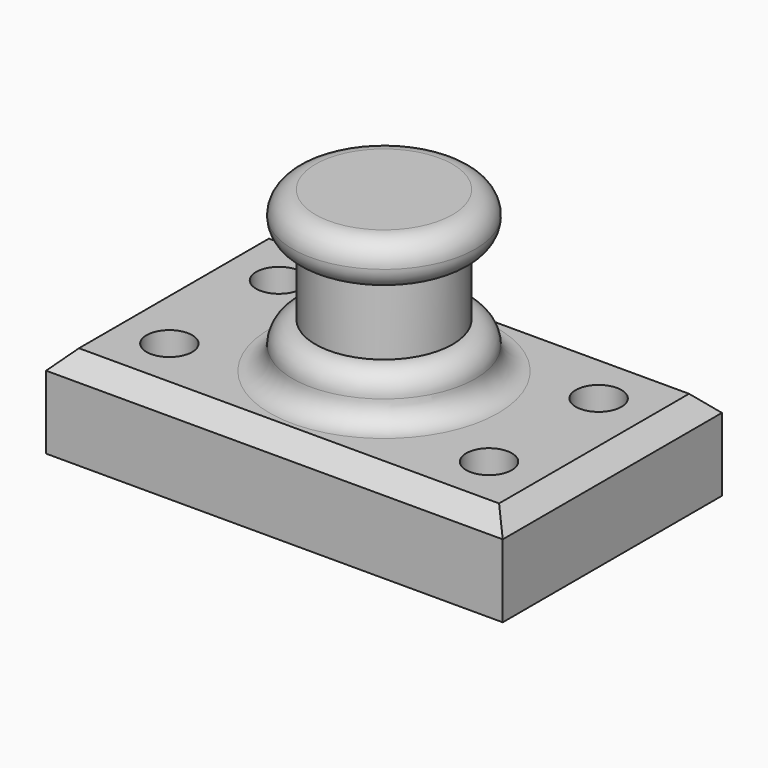
from build123d import *

# Parameters (mm, degrees)
F1_DEPTH = 25.4
F2_R     = 6.35
F3_DEPTH = 25.4
F4_W     = 25.4
F4_H     = 12.7
F6_W     = 19.05
F6_H     = 19.05
F8_W     = 25.4
F8_H     = 12.7
F11_R    = 6.34999
F12_SIZE = 5.08


# Not quite as in the source:
# - a fillet or chamfer is up to 0.001 mm smaller than in the source, because OpenCascade refuses the exact size
# - a feature of the source that left no trace in its solid (it failed there, or was rolled back) is left out


with BuildPart() as f1:
    # F0 (on Top) → F1 (new body)
    with BuildSketch(Plane.XY):
        Polygon((-63.0538856602, 38.1), (-63.5, 38.1), (-63.5, -38.1), (63.5, -38.1), (63.5, 38.1), align=None)
    extrude(amount=F1_DEPTH)

    # F2 (on face) → F3 (cut)
    with BuildSketch(Plane.XY.offset(25.4)):
        with Locations((-44.45, 19.05)):
            Circle(F2_R)
        with Locations((-44.45, -19.05)):
            Circle(F2_R)
        with Locations((44.45, 19.05)):
            Circle(F2_R)
        with Locations((44.45, -19.05)):
            Circle(F2_R)
    extrude(amount=-F3_DEPTH, mode=Mode.SUBTRACT)

    # F4 (on Front) → F5 (revolve)
    with BuildSketch(Plane.XZ):
        with Locations((12.7, 31.75)):
            Rectangle(F4_W, F4_H)
    revolve(axis=Axis((0, 0, 31.75), (0, 0, -1)))

    # F6 (on Front) → F7 (revolve)
    with BuildSketch(Plane.XZ):
        with Locations((9.525, 47.625)):
            Rectangle(F6_W, F6_H)
    revolve(axis=Axis((0, 0, 47.625), (0, 0, 1)))

    # F8 (on Front) → F9 (revolve)
    with BuildSketch(Plane.XZ):
        with Locations((12.7, 63.5)):
            Rectangle(F8_W, F8_H)
    revolve(axis=Axis((0, 0, 63.5), (0, 0, 1)))

    # F11 (radius 6.35 in the source; OpenCascade refuses exactly that, so slightly less here)
    f11_edges = [f1.edges().sort_by_distance(p)[0] for p in [
        (-25.4, 0, 69.85),
        (-25.4, 0, 38.1),
        (-25.4, 0, 57.15),
        (-25.4, 0, 25.4),
        (25.4, 0, 31.75),
    ]]
    fillet(f11_edges, radius=F11_R)

    # F12
    f12_edges = [f1.edges().sort_by_distance(p)[0] for p in [
        (-63.5, 0, 25.4),
        (0, 38.1, 25.4),
        (0, -38.1, 25.4),
        (63.5, 0, 25.4),
    ]]
    chamfer(f12_edges, length=F12_SIZE)


solid = f1.part
